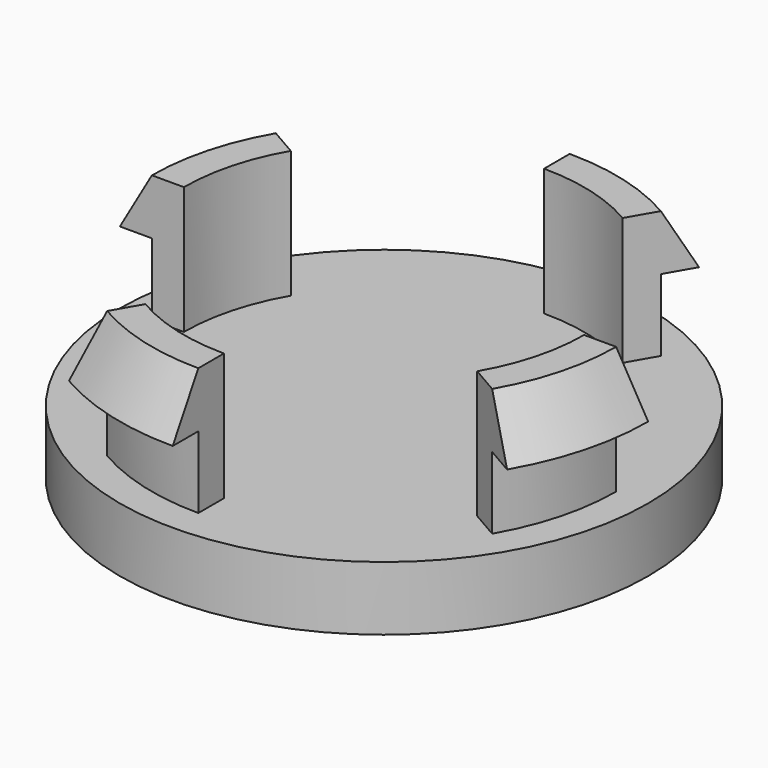
from build123d import *

# Parameters (mm, degrees)
F1_ANGLE = 30
F2_COUNT = 4


with BuildPart() as f1:
    # F0 (on Front) → F1 (revolve)
    with BuildSketch(Plane.XZ):
        Polygon((7.366, 2.032), (7.366, 4.318), (8.382, 4.318), (7.366, 6.0777636205), (6.35, 6.0777636205), (6.35, 2.032), align=None)
    revolve(axis=Axis((0, 0, 1.016), (0, 0, -1)), revolution_arc=F1_ANGLE)


with BuildPart() as f2_1:
    # F2: instance of F1
    add(f1.part.rotate(Axis((0, 0, 1.016), (0, 0, -1)), 1 * 360 / F2_COUNT))


with BuildPart() as f2_2:
    # F2: instance of F1
    add(f1.part.rotate(Axis((0, 0, 1.016), (0, 0, -1)), 2 * 360 / F2_COUNT))


with BuildPart() as f2_3:
    # F2: instance of F1
    add(f1.part.rotate(Axis((0, 0, 1.016), (0, 0, -1)), 3 * 360 / F2_COUNT))


with BuildPart() as f1_1:
    add(f1.part)

    add(f2_1.part)  # F3 merges F2_1

    add(f2_2.part)  # F3 merges F2_2

    add(f2_3.part)  # F3 merges F2_3
    # F0 (on Front) → F3 (revolve)
    with BuildSketch(Plane.XZ):
        Polygon((8.382, 2.032), (7.366, 2.032), (6.35, 2.032), (0, 2.032), (0, 0), (8.382, 0), align=None)
    revolve(axis=Axis((0, 0, 1.016), (0, 0, -1)))


solid = f1_1.part
